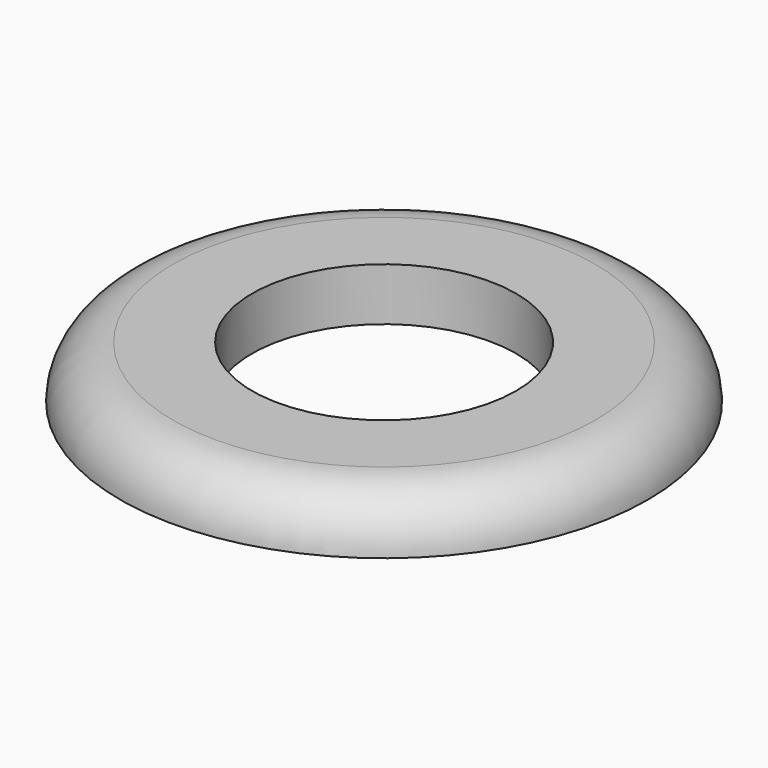
from build123d import *

# Parameters (mm, degrees)
F0_R     = 10
F1_DEPTH = 2
F2_R     = 1.99999
F3_R     = 5
F4_DEPTH = 25


# Not quite as in the source:
# - a fillet or chamfer is up to 0.001 mm smaller than in the source, because OpenCascade refuses the exact size


with BuildPart() as f1:
    # F0 (on Top) → F1 (new body)
    with BuildSketch(Plane.XY):
        Circle(F0_R)
    extrude(amount=-F1_DEPTH)

    # F2 (radius 2 in the source; OpenCascade refuses exactly that, so slightly less here)
    f2_edges = [f1.edges().sort_by_distance(p)[0] for p in [
        (-10, 0, 0),
    ]]
    fillet(f2_edges, radius=F2_R)

    # F3 (on face) → F4 (cut)
    with BuildSketch(Plane.XY):
        Circle(F3_R)
    extrude(amount=-F4_DEPTH, mode=Mode.SUBTRACT)


solid = f1.part
